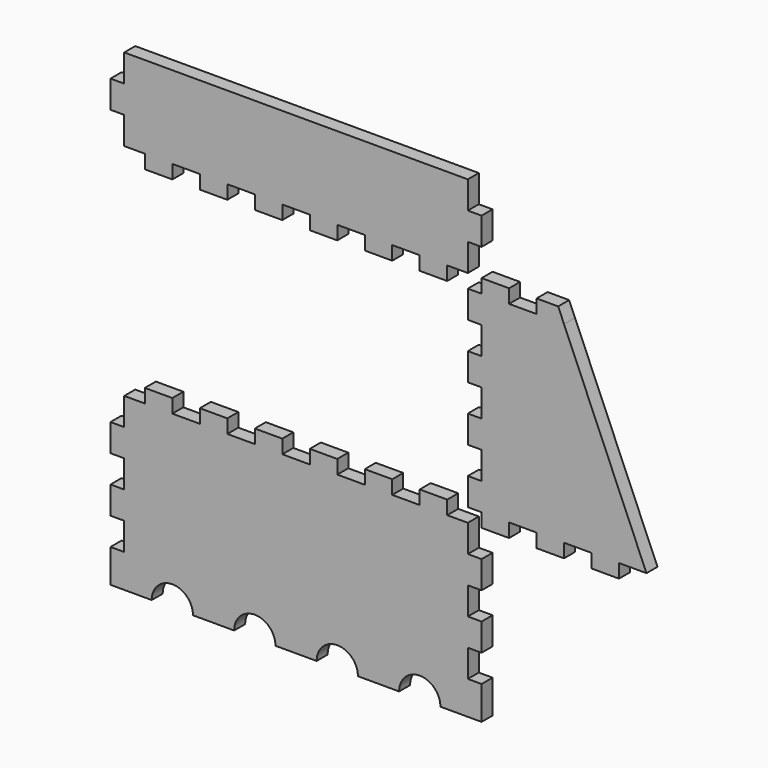
from build123d import *

# Parameters (mm, degrees)
F1_DEPTH = 10


# Not quite as in the source:
# - a feature names something its author has since deleted; it is built from what else it names


with BuildPart() as f1:
    # F0 (on Front) → F1 (new body)
    with BuildSketch(Plane.XZ):
        with BuildLine():
            Line((135, -100), (135, -110))
            Line((135, -110), (115, -110))
            Line((115, -110), (115, -100))
            Line((115, -100), (95, -100))
            Line((95, -100), (95, -110))
            Line((95, -110), (75, -110))
            Line((75, -110), (75, -100))
            Line((75, -100), (55, -100))
            Line((55, -100), (55, -110))
            Line((55, -110), (35, -110))
            Line((35, -110), (35, -100))
            Line((35, -100), (15, -100))
            Line((15, -100), (15, -110))
            Line((15, -110), (0, -110))
            Line((0, -110), (0, -130))
            Line((0, -130), (-10, -130))
            Line((-10, -130), (-10, -150))
            Line((-10, -150), (0, -150))
            Line((0, -150), (0, -170))
            Line((0, -170), (-10, -170))
            Line((-10, -170), (-10, -190))
            Line((-10, -190), (0, -190))
            Line((0, -190), (0, -210))
            Line((0, -210), (-10, -210))
            Line((-10, -210), (-10, -234.2857142857))
            Line((-10, -234.2857142857), (19.9729451345, -234.2857142857))
            ThreePointArc((19.9729451345, -234.2857142857), (34.9898544254, -219.2712298368), (50.0067637164, -234.2857142857))
            Line((50.0067637164, -234.2857142857), (79.9797088509, -234.2857142857))
            ThreePointArc((79.9797088509, -234.2857142857), (94.9966181418, -219.2712298368), (110.0135274328, -234.2857142857))
            Line((110.0135274328, -234.2857142857), (139.9864725672, -234.2857142857))
            ThreePointArc((139.9864725672, -234.2857142857), (155.0033818582, -219.2712298368), (170.0202911491, -234.2857142857))
            Line((170.0202911491, -234.2857142857), (199.9932362836, -234.2857142857))
            ThreePointArc((199.9932362836, -234.2857142857), (215.0101455746, -219.2712298368), (230.0270548655, -234.2857142857))
            Line((230.0270548655, -234.2857142857), (260, -234.2857142857))
            Line((260, -234.2857142857), (260, -210))
            Line((260, -210), (250, -210))
            Line((250, -210), (250, -190))
            Line((250, -190), (260, -190))
            Line((260, -190), (260, -170))
            Line((260, -170), (250, -170))
            Line((250, -170), (250, -150))
            Line((250, -150), (260, -150))
            Line((260, -150), (260, -130))
            Line((260, -130), (250, -130))
            Line((250, -130), (250, -110))
            Line((250, -110), (235, -110))
            Line((235, -110), (235, -100))
            Line((235, -100), (215, -100))
            Line((215, -100), (215, -110))
            Line((215, -110), (195, -110))
            Line((195, -110), (195, -100))
            Line((195, -100), (175, -100))
            Line((175, -100), (175, -110))
            Line((175, -110), (155, -110))
            Line((155, -110), (155, -100))
            Line((155, -100), (135, -100))
        make_face()
    extrude(amount=-F1_DEPTH)


with BuildPart() as f1b:
    # F0 (on Front) → F1, piece 2 (new body)
    with BuildSketch(Plane.XZ):
        Polygon((260, -100), (260, -110), (280, -110), (280, -100), (300, -100), (300, -110), (320, -110), (320, -100), (340, -100), (340, -110), (360, -110), (360, -100), (380, -100), (320, 40), (315.7142857143, 50), (300, 50), (300, 40), (280, 40), (280, 50), (260, 50), (260, 40), (250, 40), (250, 20), (260, 20), (260, 0), (250, 0), (250, -20), (260, -20), (260, -40), (250, -40), (250, -60), (260, -60), (260, -80), (250, -80), (250, -100), align=None)
    extrude(amount=-F1_DEPTH)


with BuildPart() as f1c:
    # F0 (on Front) → F1, piece 3 (new body)
    with BuildSketch(Plane.XZ):
        Polygon((235, 50), (250, 50), (250, 70), (260, 70), (260, 90), (250, 90), (250, 110), (0, 110), (0, 90), (-10, 90), (-10, 70), (0, 70), (0, 50), (15, 50), (15, 40), (35, 40), (35, 50), (55, 50), (55, 40), (75, 40), (75, 50), (95, 50), (95, 40), (115, 40), (115, 50), (135, 50), (135, 40), (155, 40), (155, 50), (175, 50), (175, 40), (195, 40), (195, 50), (215, 50), (215, 40), (235, 40), align=None)
    extrude(amount=-F1_DEPTH)


solid = Compound([f1.part, f1b.part, f1c.part])
